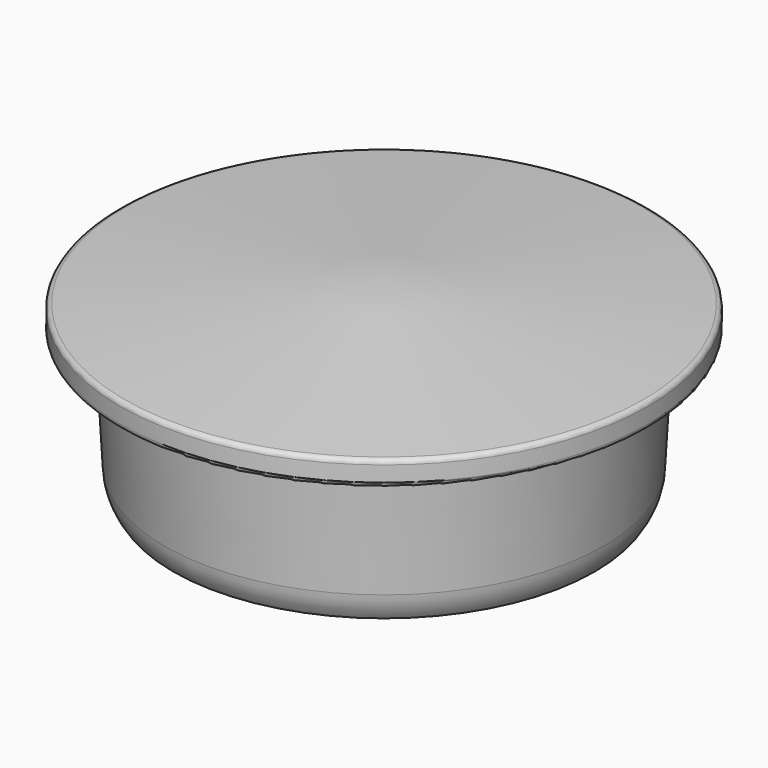
from build123d import *

# Parameters (mm, degrees)
F2_R = 0.5


# Not quite as in the source:
# - a fillet or chamfer that OpenCascade refuses, or shapes differently, is made with other operations: its cross-section is extruded or revolved along the edge and cut away or added


with BuildPart() as f1:
    # F0 (on Front) → F1 (revolve)
    with BuildSketch(Plane.XZ):
        Polygon((23, -15), (23.8, 0), (22.05, 0), (22.2, -15), align=None)
        Polygon((22.05, 0), (23.8, 0), (27.8, 0), (27.8, 2.6), (0, 5), (0, 2.5), align=None)
    revolve(axis=Axis((0, 0, 3.75), (0, 0, -1)))

    # F2
    f2_edges = [f1.edges().sort_by_distance(p)[0] for p in [
        (-27.8, 0, 2.6),
        (-27.8, 0, 0),
    ]]
    fillet(f2_edges, radius=F2_R)

    # F3: fillet of radius 5 on 2 edges, made by hand

    # F3_s1 → F3_t2 (revolve)
    with BuildSketch(Plane.XZ):
        with BuildLine():
            ThreePointArc((22.0942018316, -4.4201831603), (20.8071251, -1.121142431), (17.6577363633, 0.4979890745))
            Line((17.6577363633, 0.4979890745), (17.6690020543, 0.5973524692))
            Line((17.6690020543, 0.5973524692), (22.1491109637, 0.0894036132))
            Line((22.1491109637, 0.0894036132), (22.194196832, -4.4191832103))
            Line((22.194196832, -4.4191832103), (22.0942018316, -4.4201831603))
        make_face()
    revolve(axis=Axis((0, 0, 0), (0, 0, -1)))

    # F3_s3 → F3_t4 (revolve, cut)
    with BuildSketch(Plane.XZ):
        with BuildLine():
            ThreePointArc((23.1421216086, -12.335219838), (22.8632741638, -13.7355661287), (22.2, -15))
            Line((22.2, -15), (22.2810156483, -15.0586213675))
            ThreePointArc((22.2810156483, -15.0586213675), (22.6, -15.1), (23, -15.1))
            Line((23, -15.1), (23.0998580805, -15.0053257643))
            Line((23.0998580805, -15.0053257643), (23.2419796891, -12.3405456023))
            Line((23.2419796891, -12.3405456023), (23.1421216086, -12.335219838))
        make_face()
    revolve(axis=Axis((0, 0, -15), (0, 0, -1)), mode=Mode.SUBTRACT)


solid = f1.part
